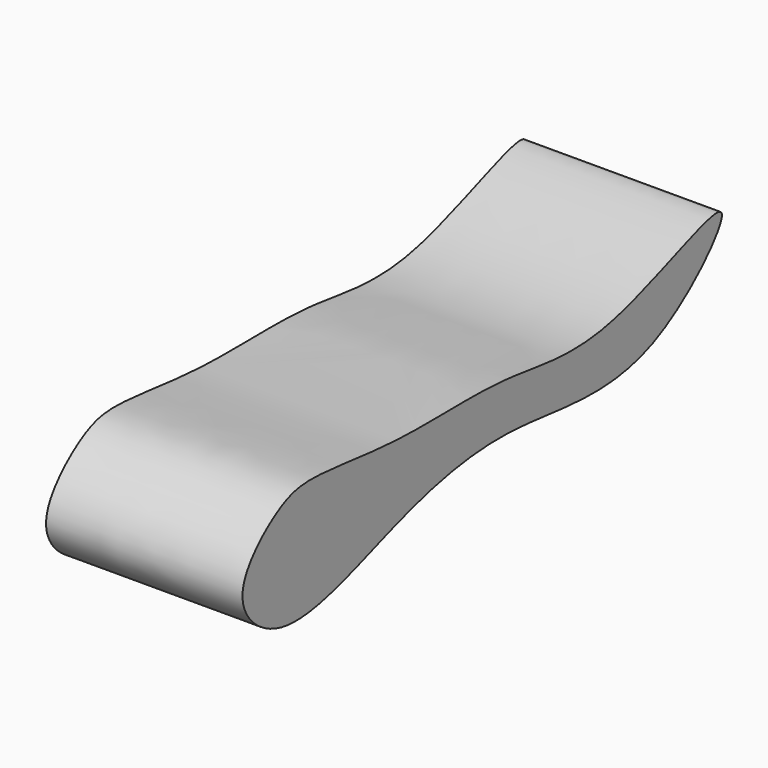
from build123d import *

# Parameters (mm, degrees)
F4_DEPTH = 24.3


# Not quite as in the source:
# - the program builds the solid bodies; features that only make, move or delete a surface that nothing else refers to are left out


with BuildPart() as f4:
    # F3 (on offset) → F4 (new body)
    with BuildSketch(Plane.YZ.offset(-106.4)):
        with BuildLine():
            add(Edge.make_bspline(
                [(-26.8738996238, -33.3181507885), (-31.7985846948, -33.0810381629), (-39.6753658358, -31.7567749517), (-45.184545597, -32.808220076), (-53.5799036524, -40.4378318936), (-44.1872605114, -49.6540103639), (-26.1012684804, -41.3512050956), (-8.6665931873, -38.1613860037), (11.9420613326, -43.6179151391), (30.3358664671, -23.4107638312), (4.7288171389, -36.8274718367), (-9.5991098249, -32.6782708038), (-21.2732285966, -33.5878106335), (-26.8738996238, -33.3181507885)],
                knots=[0, 0, 0, 0, 0.0872592718, 0.1449460796, 0.216834693, 0.2877023398, 0.3922271061, 0.4960314182, 0.6082815771, 0.7002030135, 0.8015261827, 0.9007631009, 1, 1, 1, 1], degree=3))
        make_face()
    extrude(amount=-F4_DEPTH)


with BuildPart() as f4_1:
    # F5: moved
    add(f4.part.moved(Location((0, 0, 37.8))))


solid = f4_1.part
